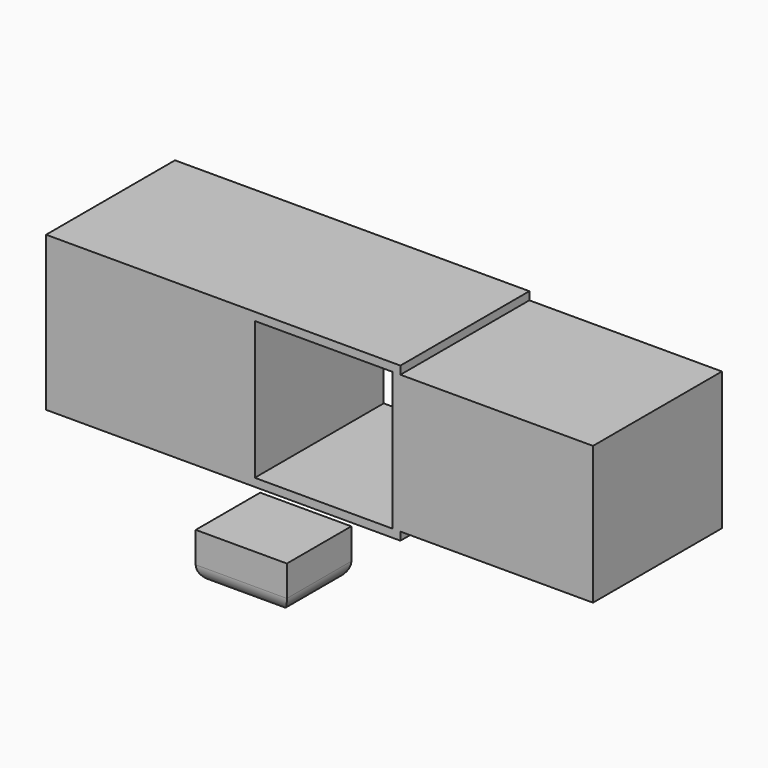
from build123d import *

# Parameters (mm, degrees)
F0_W        = 111.691813916
F0_H        = 48.596679233
F1_DEPTH    = 25.4
F0_W_2      = 28.7284236401
F0_H_2      = 14.766946435
F2_T        = -2.54
F3_DEPTH    = 63.246
F4_DEPTH    = 25.4
F5_T        = 2.54
F5_T3_DEPTH = 55.88
F6_R        = 5.08


# Not quite as in the source:
# - a shell that OpenCascade refuses in one call is made with other operations: the cavity is built on its own and cut out


with BuildPart() as f1:
    # F0 (on Front) → F1 (new body)
    with BuildSketch(Plane.XZ):
        with Locations((-17.4518469721, 34.500957001)):
            Rectangle(F0_W, F0_H)
    extrude(amount=F1_DEPTH)

    # F2
    f2_openings = [f1.faces().sort_by_distance(p)[0] for p in [
        (-17.451847, -25.4, 34.500957),
        (-17.451847, 0, 34.500957),
    ]]
    offset(amount=F2_T, openings=f2_openings)

    # F3 (add): faces of the model
    f3_faces = [f1.faces().sort_by_distance(p)[0] for p in [
        (-70.7577539301, -12.7, 34.500957001),
        (35.8540599859, -12.7, 34.500957001),
    ]]
    extrude(f3_faces, amount=F3_DEPTH, dir=(1, 0, 0))

    # F4 (add): a face of the model
    f4_faces = [f1.faces().sort_by_distance(p)[0] for p in [
        (36.602897138, -25.4, 57.5292966175),
    ]]
    extrude(f4_faces, amount=F4_DEPTH)

    # F5: shell of thickness 2.54, made by hand


with BuildPart() as f1b:
    # F0 (on Front) → F1, piece 2 (new body)
    with BuildSketch(Plane.XZ):
        with Locations((-32.0845479146, -32.0845469832)):
            Rectangle(F0_W_2, F0_H_2)
    extrude(amount=F1_DEPTH)

    # F6
    f6_edges = [f1b.edges().sort_by_distance(p)[0] for p in [
        (-46.44876, -12.7, -39.46802),
        (-17.720336, -12.7, -39.46802),
        (-32.084548, 0, -39.46802),
        (-32.084548, -25.4, -39.46802),
    ]]
    fillet(f6_edges, radius=F6_R)


with BuildPart() as f5_core1:
    # F5_t2: copy of F1
    add(f1.part)

    # the walls: a layer under each face that stays
    f5_faces = [f5_core1.faces().sort_by_distance(p)[0] for p in [
        (-17.4518469721, -25.4, 58.7992966175),
        (-7.5117539301, -25.4, 34.500957001),
        (14.1711530279, -25.4, 12.7426173845),
        (35.8540599859, -25.4, 34.500957001),
        (14.1711530279, -25.4, 56.2592966175),
        (68.7470599859, -25.4, 56.2592966175),
        (99.1000599859, -25.4, 34.500957001),
        (68.7470599859, -25.4, 12.7426173845),
        (38.3940599859, -25.4, 11.4726173845),
        (-17.4518469721, -25.4, 10.2026173845),
        (-73.2977539301, -25.4, 34.500957001),
        (-44.5647849441, -50.8, 18.3020639233),
        (38.3940599859, -25.4, 57.5292966175),
    ]]
    thicken(f5_faces, amount=-F5_T, mode=Mode.SUBTRACT)

    # F5_s4 → F5_t3 (cut)
    with BuildSketch(Plane.XZ.offset(-2.54)):
        Polygon((-7.4863539301, 56.2338966175), (-10.0517539301, 56.2592966175), (-10.0517539301, 58.7992966175), (-7.5117539301, 58.7992966175), align=None)
        Polygon((-7.4863539301, 12.7680173845), (-10.0517539301, 12.7426173845), (-10.0517539301, 10.2026173845), (-7.5117539301, 10.2026173845), align=None)
        Polygon((35.8286599859, 12.7680173845), (35.8540599859, 10.2026173845), (38.3940599859, 10.2026173845), (38.3940599859, 12.7426173845), align=None)
        Polygon((35.8286599859, 56.2338966175), (38.3940599859, 56.2592966175), (38.3940599859, 58.7992966175), (35.8540599859, 58.7992966175), align=None)
        Polygon((38.4194599859, 56.2846966175), (38.3940599859, 53.7192966175), (35.8540599859, 53.7192966175), (35.8540599859, 56.2592966175), align=None)
        Polygon((38.4194599859, 12.7172173845), (38.3940599859, 15.2826173845), (35.8540599859, 15.2826173845), (35.8540599859, 12.7426173845), align=None)
    extrude(amount=F5_T3_DEPTH, mode=Mode.SUBTRACT)


with BuildPart() as f1_1:
    add(f1.part)

    # what is left inside the walls is the cavity
    f5_cavity = [f5_core1.part.solids().sort_by_distance(p)[0] for p in [
        (77.171393, -24.13, 53.693897),
        (-40.404754, -32.173333, 56.233897),
    ]]
    add(f5_cavity, mode=Mode.SUBTRACT)


solid = Compound([f1b.part, f1_1.part])
